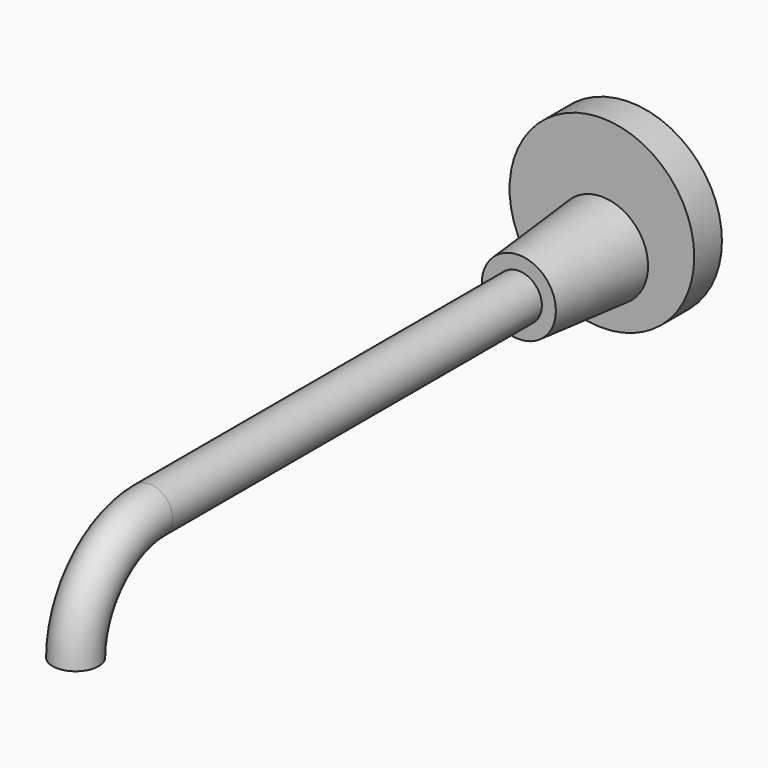
from build123d import *

# Parameters (mm, degrees)
F0_R     = 50.8
F1_DEPTH = 19.05
F2_R     = 25.4
F3_DEPTH = 57.15
F3_TAPER = 5
F4_R     = 12.7
F5_DEPTH = 254
F6_R     = 12.7


# Not quite as in the source:
# - the program builds the solid bodies; features that only make, move or delete a surface that nothing else refers to are left out


with BuildPart() as f1:
    # F0 (on Front) → F1 (new body)
    with BuildSketch(Plane.XZ):
        Circle(F0_R)
    extrude(amount=F1_DEPTH)

    # F2 (on face) → F3 (join)
    with BuildSketch(Plane.XZ.offset(19.05)):
        with Locations((0, -12.7)):
            Circle(F2_R)
    extrude(amount=F3_DEPTH, taper=F3_TAPER)

    # F4 (on face) → F5 (join)
    with BuildSketch(Plane.XZ.offset(76.2)):
        with Locations((0, -12.7)):
            Circle(F4_R)
    extrude(amount=F5_DEPTH)

    # F8: sweep along a path in F7
    with BuildLine(Plane.YZ) as f8_path:
        ThreePointArc((-330.2, -12.7), (-366.1210244843, -27.5789755157), (-381, -63.5))
    # F6 (on face) → F8 (sweep)
    with BuildSketch(Plane.XZ.offset(330.2)):
        with Locations((0, -12.7)):
            Circle(F6_R)
    sweep(path=f8_path.line)


solid = f1.part
